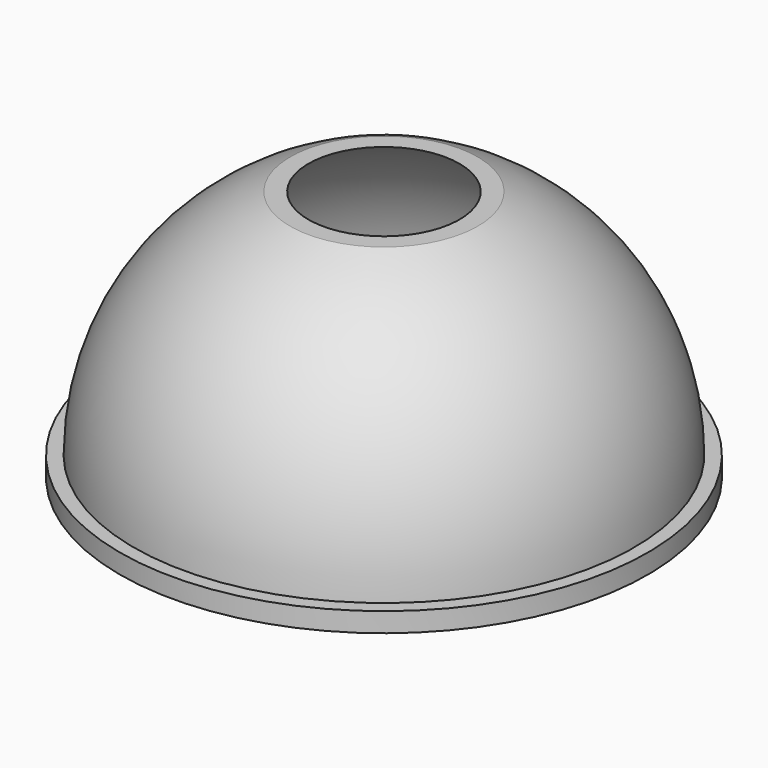
from build123d import *

# Parameters (mm, degrees)
F3_T = -1
F4_T = 0.2


# Not quite as in the source:
# - a shell that OpenCascade refuses in one call is made with other operations: the cavity is built on its own and cut out


with BuildPart() as f2:
    # F0 (on Right) → F2 (revolve)
    with BuildSketch(Plane.YZ):
        with BuildLine():
            Line((15, 37.0809924355), (0, 37.0809924355))
            Line((0, 37.0809924355), (0, 0))
            Line((0, 0), (0, -3.1108935364))
            Line((0, -3.1108935364), (42.2, -3.1108935364))
            Line((42.2, -3.1108935364), (42.2, 0))
            Line((42.2, 0), (40, 0))
            ThreePointArc((40, 0), (33.1662479036, 22.360679775), (15, 37.0809924355))
        make_face()
    revolve(axis=Axis((0, 0, 9.5782782882), (0, 0, -1)))

    # F3
    f3_openings = [f2.faces().sort_by_distance(p)[0] for p in [
        (0, 0, 37.080992),
        (0, 0, -3.110894),
    ]]
    offset(amount=F3_T, openings=f3_openings, kind=Kind.INTERSECTION)

    # F4: shell of thickness 0.2, made by hand


with BuildPart() as f4_core1:
    # F4_t2: copy of F2
    add(f2.part)

    # the walls: a layer under each face that stays
    f4_faces = [f4_core1.faces().sort_by_distance(p)[0] for p in [
        (0, -42.2, -1.5554467682),
        (-11.2533333333, -39.3866666667, 0),
        (0, -33.1662479036, 22.360679775),
        (-10, -10, 37.0809924355),
        (0, -31.8525104905, 22.5037235909),
        (-20.3185185185, -36.925, -3.1108935364),
        (-10.9866666667, -38.4533333333, -1),
    ]]
    thicken(f4_faces, amount=-F4_T, mode=Mode.SUBTRACT)

    # F4_s3 → F4_t4 (revolve, cut)
    with BuildSketch(Plane.YZ):
        Polygon((40.002, 0.002), (40, -0.2), (39.8, -0.2), (39.8, 0), align=None)
    revolve(axis=Axis((0, 0, 0), (0, 0, -1)), mode=Mode.SUBTRACT)


with BuildPart() as f2_1:
    add(f2.part)

    # what is left inside the walls is the cavity
    f4_cavity = [f4_core1.part.solids().sort_by_distance(p)[0] for p in [
        (0, -36.186898, 15.076644),
    ]]
    add(f4_cavity, mode=Mode.SUBTRACT)


solid = f2_1.part
